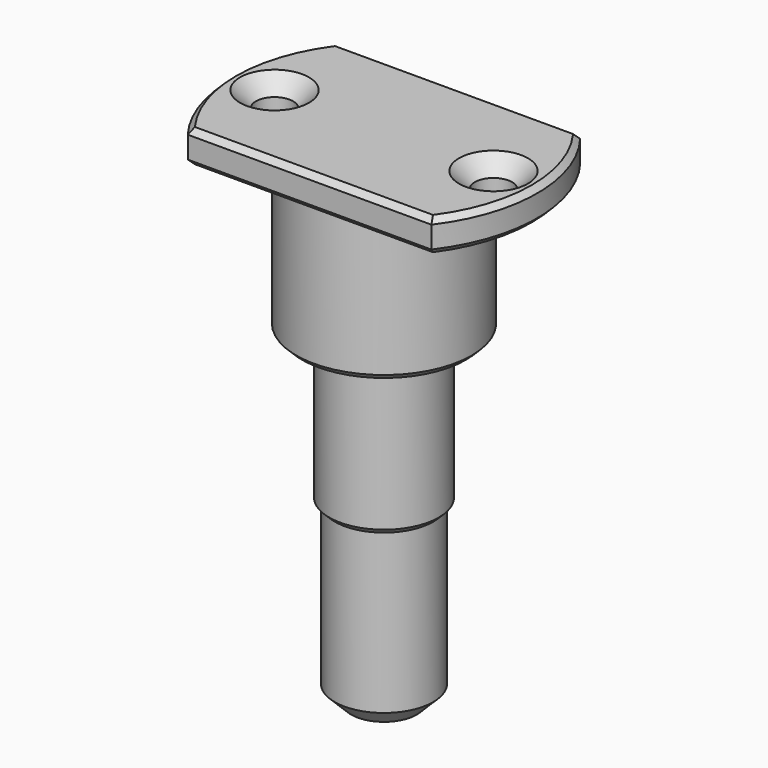
from build123d import *

# Parameters (mm, degrees)
F1_DEPTH       = 3
F2_SIZE        = 0.5
F4_D           = 3.4
F4_CSINK_D     = 6.3
F4_CSINK_ANGLE = 90
F5_R           = 8
F6_DEPTH       = 13
F7_R           = 5
F8_DEPTH       = 14
F9_R           = 4.5
F10_DEPTH      = 16
F11_SIZE       = 1.5
F12_SIZE       = 0.49999


# Not quite as in the source:
# - a fillet or chamfer is up to 0.001 mm smaller than in the source, because OpenCascade refuses the exact size


with BuildPart() as f1:
    # F0 (on Top) → F1 (new body)
    with BuildSketch(Plane.XY):
        with BuildLine():
            Line((11.1242977306, 8.5), (-11.1242977306, 8.5))
            ThreePointArc((-11.1242977306, 8.5), (-14, 0), (-11.1242977306, -8.5))
            Line((-11.1242977306, -8.5), (11.1242977306, -8.5))
            ThreePointArc((11.1242977306, -8.5), (14, 0), (11.1242977306, 8.5))
        make_face()
    extrude(amount=F1_DEPTH)

    # F2
    f2_edges = [f1.edges().sort_by_distance(p)[0] for p in [
        (0, -8.5, 3),
        (14, 0, 3),
        (0, 8.5, 3),
        (-14, 0, 3),
        (0, -8.5, 0),
        (14, 0, 0),
        (0, 8.5, 0),
        (-14, 0, 0),
    ]]
    chamfer(f2_edges, length=F2_SIZE)

    # F4 (through all)
    with Locations(Plane.XY.offset(3)):
        with Locations((-10, 0), (10, 0)):
            CounterSinkHole(F4_D / 2, F4_CSINK_D / 2, counter_sink_angle=F4_CSINK_ANGLE)

    # F5 (on face) → F6 (join)
    with BuildSketch(Plane(origin=(0, 0, 0), x_dir=(1, 0, 0), z_dir=(0, 0, -1))):
        Circle(F5_R)
    extrude(amount=F6_DEPTH)

    # F7 (on face) → F8 (join)
    with BuildSketch(Plane(origin=(0, 0, -13), x_dir=(1, 0, 0), z_dir=(0, 0, -1))):
        Circle(F7_R)
    extrude(amount=F8_DEPTH)

    # F9 (on face) → F10 (join)
    with BuildSketch(Plane(origin=(0, 0, -27), x_dir=(1, 0, 0), z_dir=(0, 0, -1))):
        Circle(F9_R)
    extrude(amount=F10_DEPTH)

    # F11
    f11_edges = [f1.edges().sort_by_distance(p)[0] for p in [
        (-4.5, 0, -43),
    ]]
    chamfer(f11_edges, length=F11_SIZE)

    # F12 (size 0.5 in the source; OpenCascade refuses exactly that, so slightly less here)
    f12_edges = [f1.edges().sort_by_distance(p)[0] for p in [
        (-5, 0, -27),
        (-8, 0, -13),
    ]]
    chamfer(f12_edges, length=F12_SIZE)


solid = f1.part
